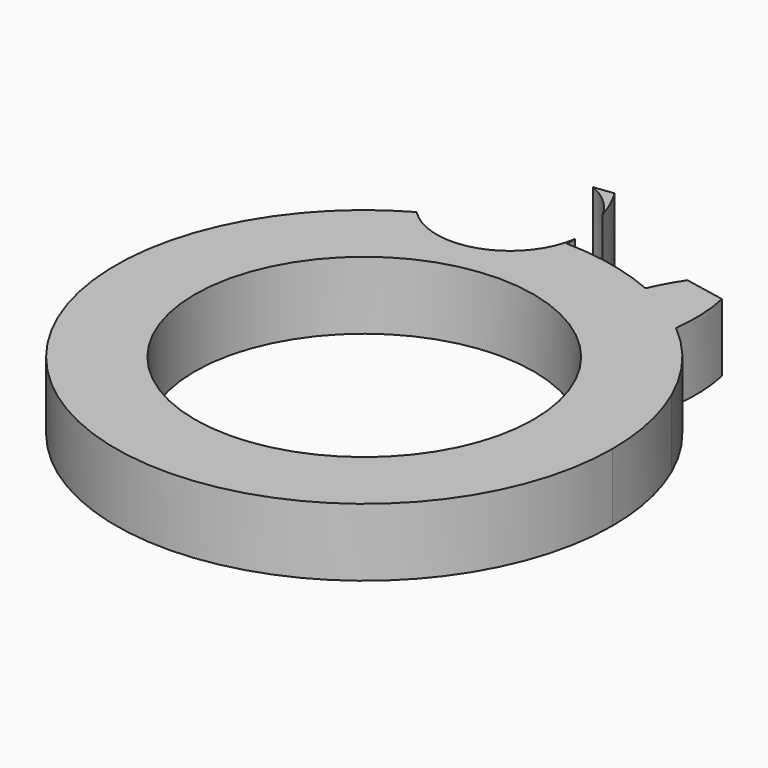
from build123d import *

# Parameters (mm, degrees)
F2_R     = 2.5
F3_DEPTH = 1


# Not quite as in the source:
# - a feature of the source that left no trace in its solid (it failed there, or was rolled back) is left out


with BuildPart() as f3:
    # F2 (on Top) → F3 (new body)
    with BuildSketch(Plane.XY):
        with BuildLine():
            ThreePointArc((-1.7882578064, 3.2010277197), (-1.8557342421, -3.1623875264), (3.6666666667, 0))
            ThreePointArc((3.6666666667, 0), (3.5899247335, 0.746247179), (3.3629112928, 1.461257021))
            ThreePointArc((3.3629112928, 1.461257021), (2.9368456583, 2.1953090953), (2.353421422, 2.8117347056))
            ThreePointArc((2.353421422, 2.8117347056), (1.9271816651, 3.1193613568), (1.4613338593, 3.3628779038))
            ThreePointArc((1.4613338593, 3.3628779038), (0.7754810346, 3.5837234281), (0.0596824548, 3.6661809078))
            ThreePointArc((0.0596824548, 3.6661809078), (0.0418652156, 3.6664276548), (0.0240469876, 3.6665878125))
            ThreePointArc((0.0240469876, 3.6665878125), (-0.7484563132, 2.913546469), (-1.7882578064, 3.2010277197))
        make_face()
        Circle(F2_R, mode=Mode.SUBTRACT)
        with BuildLine():
            ThreePointArc((1.4613338593, 3.3628779038), (1.9271816651, 3.1193613568), (2.353421422, 2.8117347056))
            ThreePointArc((2.353421422, 2.8117347056), (2.3729229005, 3.2594447829), (2.3156558798, 3.7039052528))
            Line((2.3156558798, 3.7039052528), (1.7123740108, 3.8220121342))
            ThreePointArc((1.7123740108, 3.8220121342), (1.5753344373, 3.598743518), (1.4613338593, 3.3628779038))
        make_face()
        with BuildLine():
            ThreePointArc((0.0556967301, 3.8186389948), (0.0426001878, 3.7420454968), (0.0240469876, 3.6665878125))
            ThreePointArc((0.0240469876, 3.6665878125), (0.0418652156, 3.6664276548), (0.0596824548, 3.6661809078))
            ThreePointArc((0.0596824548, 3.6661809078), (0.0588018532, 3.7424390292), (0.0556967301, 3.8186389948))
        make_face()
    extrude(amount=F3_DEPTH)


with BuildPart() as f3b:
    # F2 (on Top) → F3, piece 2 (new body)
    with BuildSketch(Plane.XY):
        with BuildLine():
            Line((-0.2964174653, 4.9912059351), (-0.5855698897, 4.9560964742))
            ThreePointArc((-0.5855698897, 4.9560964742), (-0.2889775443, 4.7641459457), (-0.0699158309, 4.4869745359))
            ThreePointArc((-0.0699158309, 4.4869745359), (-0.1697989463, 4.7450950307), (-0.2964174653, 4.9912059351))
        make_face()
    extrude(amount=F3_DEPTH)


solid = Compound([f3.part, f3b.part])
